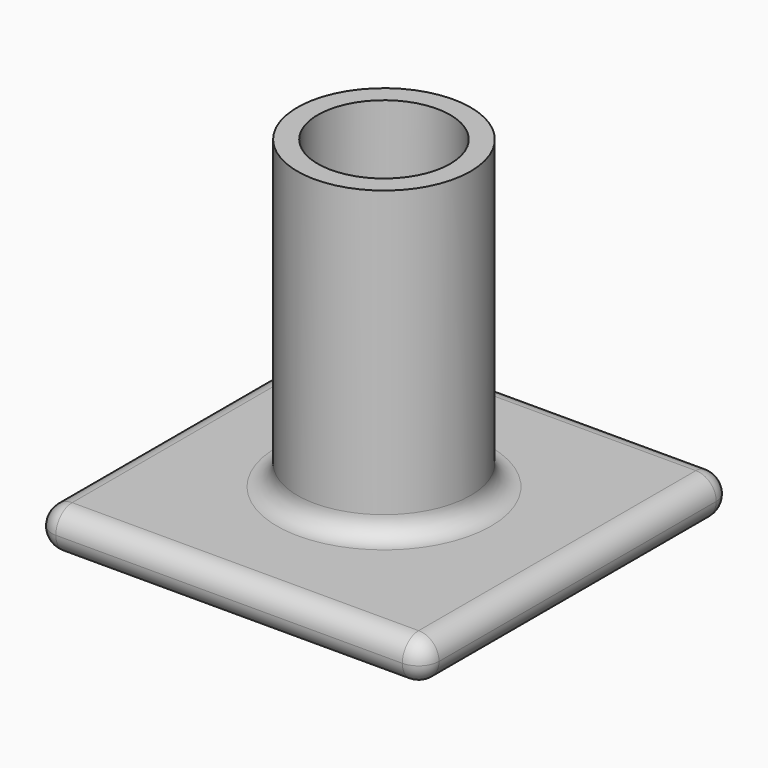
from build123d import *

# Parameters (mm, degrees)
F0_R     = 8.5
F0_R_2   = 6.5
F1_DEPTH = 30
F2_W     = 38
F2_H     = 38
F2_R     = 6.5
F3_DEPTH = 4
F4_R     = 1.99999


# Not quite as in the source:
# - a fillet or chamfer is up to 0.001 mm smaller than in the source, because OpenCascade refuses the exact size


with BuildPart() as f1:
    # F0 (on Top) → F1 (new body)
    with BuildSketch(Plane.XY):
        Circle(F0_R)
        Circle(F0_R_2, mode=Mode.SUBTRACT)
    extrude(amount=F1_DEPTH)

    # F2 (on Top) → F3 (join)
    with BuildSketch(Plane.XY):
        Rectangle(F2_W, F2_H)
        Circle(F2_R, mode=Mode.SUBTRACT)
    extrude(amount=-F3_DEPTH)

    # F4 (radius 2 in the source; OpenCascade refuses exactly that, so slightly less here)
    f4_edges = [f1.edges().sort_by_distance(p)[0] for p in [
        (0, -19, -4),
        (19, 0, -4),
        (0, 19, -4),
        (-19, 0, -4),
        (-6.5, 0, -4),
        (0, -19, 0),
        (-19, 0, 0),
        (19, 0, 0),
        (0, 19, 0),
        (-8.5, 0, 0),
        (19, 19, -2),
        (-19, 19, -2),
        (19, -19, -2),
        (-19, -19, -2),
    ]]
    fillet(f4_edges, radius=F4_R)


solid = f1.part
